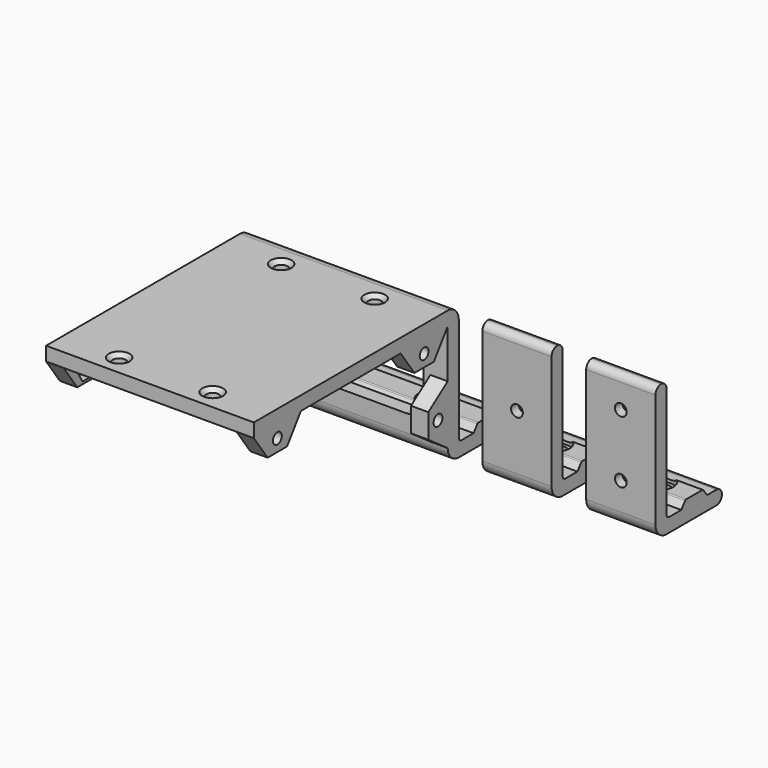
from build123d import *

# Parameters (mm, degrees)
F1_DEPTH        = 20
F2_R            = 3
F3_DEPTH        = 6
F7_D            = 3.4
F7_DEPTH        = 12
F7_CSINK_D      = 6
F7_CSINK_ANGLE  = 90
F7_TIP          = 1.0214630523
F10_DEPTH       = 20
F11_R           = 3
F12_DEPTH       = 12.5
F13_R           = 4
F14_DEPTH       = 2
F16_D           = 3.4
F16_DEPTH       = 12
F16_CSINK_D     = 6
F16_CSINK_ANGLE = 90
F16_TIP         = 1.0214630523
F19_DEPTH       = 60
F20_W           = 60
F20_H           = 70
F21_DEPTH       = 4
F22_R           = 4
F24_D           = 5.7
F25_R           = 2.85
F26_DEPTH       = 2
F28_D           = 3.7
F28_CSINK_D     = 6
F28_CSINK_ANGLE = 90
F4_R            = 4
F29_DEPTH       = 2
F31_DEPTH       = 25
F33_DEPTH       = 5
F32_R           = 1.6
F34_DEPTH       = 2.5
F40_ANGLE       = 90


with BuildPart() as f1:
    # F0 (on Right) → F1 (new body)
    with BuildSketch(Plane.YZ):
        with BuildLine():
            Line((5.35, 0), (1, 0))
            ThreePointArc((1, 0), (0.2928932188, 0.2928932188), (0, 1))
            Line((0, 1), (0, 33))
            ThreePointArc((0, 33), (-0.5857864376, 34.4142135624), (-2, 35))
            ThreePointArc((-2, 35), (-3.4142135624, 34.4142135624), (-4, 33))
            Line((-4, 33), (-4, 0))
            ThreePointArc((-4, 0), (-2.8284271247, -2.8284271247), (0, -4))
            Line((0, -4), (18, -4))
            ThreePointArc((18, -4), (19.4142135624, -3.4142135624), (20, -2))
            ThreePointArc((20, -2), (19.4142135624, -0.5857864376), (18, 0))
            Line((18, 0), (14.65, 0))
            Line((14.65, 0), (5.35, 0))
        make_face()
        with BuildLine():
            Line((6.7, 1.8), (5.35, 0))
            Line((5.35, 0), (14.65, 0))
            Line((14.65, 0), (13.3, 1.8))
            ThreePointArc((13.3, 1.8), (13.1236067977, 1.9472135955), (12.9, 2))
            Line((12.9, 2), (10, 2))
            Line((10, 2), (7.1, 2))
            ThreePointArc((7.1, 2), (6.8763932023, 1.9472135955), (6.7, 1.8))
        make_face()
    extrude(amount=F1_DEPTH)

    # F2 (on face) → F3 (cut, through all)
    with BuildSketch(Plane(origin=(0, 0, -4), x_dir=(1, 0, 0), z_dir=(0, 0, -1))):
        with Locations((10, -10)):
            Circle(F2_R)
    extrude(amount=-F3_DEPTH, mode=Mode.SUBTRACT)

    # F7
    with Locations(Plane(origin=(0, 0, 0), x_dir=(-1, 0, 0), z_dir=(0, 1, 0))):
        with Locations((-10, 26), (-10, 8)):
            CounterSinkHole(F7_D / 2, F7_CSINK_D / 2, depth=F7_DEPTH, counter_sink_angle=F7_CSINK_ANGLE)
            with Locations((0, 0, -(F7_DEPTH + F7_TIP / 2))):  # 118° drill point
                Cone(0, F7_D / 2, F7_TIP, mode=Mode.SUBTRACT)

    # F4 (on face) → F29 (cut)
    with BuildSketch(Plane.XY.offset(2)):
        with Locations((10, 10)):
            Circle(F4_R)
    extrude(amount=-F29_DEPTH, mode=Mode.SUBTRACT)


with BuildPart() as f10:
    # F9 (on offset) → F10 (new body)
    with BuildSketch(Plane.YZ.offset(-10)):
        with BuildLine():
            ThreePointArc((1, 0), (0.2928932188, 0.2928932188), (0, 1))
            Line((0, 1), (0, 33))
            ThreePointArc((0, 33), (-0.5857864376, 34.4142135624), (-2, 35))
            ThreePointArc((-2, 35), (-3.4142135624, 34.4142135624), (-4, 33))
            Line((-4, 33), (-4, 0))
            ThreePointArc((-4, 0), (-2.8284271247, -2.8284271247), (0, -4))
            Line((0, -4), (18, -4))
            ThreePointArc((18, -4), (19.4142135624, -3.4142135624), (20, -2))
            ThreePointArc((20, -2), (19.4142135624, -0.5857864376), (18, 0))
            Line((18, 0), (14.65, 0))
            Line((14.65, 0), (5.35, 0))
            Line((5.35, 0), (1, 0))
        make_face()
        with BuildLine():
            Line((6.7, 1.8), (5.35, 0))
            Line((5.35, 0), (14.65, 0))
            Line((14.65, 0), (13.3, 1.8))
            ThreePointArc((13.3, 1.8), (13.1236067977, 1.9472135955), (12.9, 2))
            Line((12.9, 2), (10, 2))
            Line((10, 2), (7.1, 2))
            ThreePointArc((7.1, 2), (6.8763932023, 1.9472135955), (6.7, 1.8))
        make_face()
    extrude(amount=-F10_DEPTH)

    # F11 (on face) → F12 (cut, symmetric)
    with BuildSketch(Plane.XY):
        with Locations((-20, 10)):
            Circle(F11_R)
    extrude(amount=F12_DEPTH, both=True, mode=Mode.SUBTRACT)

    # F13 (on face) → F14 (cut)
    with BuildSketch(Plane.XY.offset(2)):
        with Locations((-20, 10)):
            Circle(F13_R)
    extrude(amount=-F14_DEPTH, mode=Mode.SUBTRACT)

    # F16
    with Locations(Plane(origin=(0, 0, 0), x_dir=(-1, 0, 0), z_dir=(0, 1, 0))):
        with Locations((20, 16)):
            CounterSinkHole(F16_D / 2, F16_CSINK_D / 2, depth=F16_DEPTH, counter_sink_angle=F16_CSINK_ANGLE)
            with Locations((0, 0, -(F16_DEPTH + F16_TIP / 2))):  # 118° drill point
                Cone(0, F16_D / 2, F16_TIP, mode=Mode.SUBTRACT)


with BuildPart() as f19:
    # F18 (on offset) → F19 (new body)
    with BuildSketch(Plane.YZ.offset(-40)):
        with BuildLine():
            Line((0, 35.0000039041), (-4, 35.0000039041))
            Line((-4, 35.0000039041), (-4, 0))
            ThreePointArc((-4, 0), (-2.8284271247, -2.8284271247), (0, -4))
            Line((0, -4), (18, -4))
            ThreePointArc((18, -4), (19.4142135624, -3.4142135624), (20, -2))
            ThreePointArc((20, -2), (19.4142135624, -0.5857864376), (18, 0))
            Line((18, 0), (14.65, 0))
            Line((14.65, 0), (5.35, 0))
            Line((5.35, 0), (1, 0))
            ThreePointArc((1, 0), (0.2928932188, 0.2928932188), (0, 1))
            Line((0, 1), (0, 35.0000039041))
        make_face()
        with BuildLine():
            Line((6.7, 1.8), (5.35, 0))
            Line((5.35, 0), (14.65, 0))
            Line((14.65, 0), (13.3, 1.8))
            ThreePointArc((13.3, 1.8), (13.1236067977, 1.9472135955), (12.9, 2))
            Line((12.9, 2), (10, 2))
            Line((10, 2), (7.1, 2))
            ThreePointArc((7.1, 2), (6.8763932023, 1.9472135955), (6.7, 1.8))
        make_face()
    extrude(amount=-F19_DEPTH)

    # F20 (on face) → F21 (join)
    with BuildSketch(Plane.XY.offset(35.0000039041)):
        with Locations((-70, -39)):
            Rectangle(F20_W, F20_H)
    extrude(amount=-F21_DEPTH)

    # F22
    f22_edges = [f19.edges().sort_by_distance(p)[0] for p in [
        (-70, 0, 35.000004),
    ]]
    fillet(f22_edges, radius=F22_R)

    # F24 (through all)
    with Locations(Plane(origin=(0, 0, -4), x_dir=(1, 0, 0), z_dir=(0, 0, -1))):
        with Locations((-85, -10), (-55, -10)):
            Hole(F24_D / 2)

    # F25 (on face) → F26 (cut, through all)
    with BuildSketch(Plane.XY.offset(2)):
        with BuildLine():
            ThreePointArc((-81.5590698932, 7.1), (-80.7730516042, 8.4563331772), (-80.5, 10))
            ThreePointArc((-80.5, 10), (-80.7730516042, 11.5436668228), (-81.5590698932, 12.9))
            Line((-81.5590698932, 12.9), (-88.4409301068, 12.9))
            ThreePointArc((-88.4409301068, 12.9), (-89.5, 10), (-88.4409301068, 7.1))
            Line((-88.4409301068, 7.1), (-81.5590698932, 7.1))
        make_face()
        with Locations((-85, 10)):
            Circle(F25_R, mode=Mode.SUBTRACT)
        with BuildLine():
            Line((-51.5590698932, 12.9), (-58.4409301068, 12.9))
            ThreePointArc((-58.4409301068, 12.9), (-59.5, 10), (-58.4409301068, 7.1))
            Line((-58.4409301068, 7.1), (-51.5590698932, 7.1))
            ThreePointArc((-51.5590698932, 7.1), (-50.7730516042, 8.4563331772), (-50.5, 10))
            ThreePointArc((-50.5, 10), (-50.7730516042, 11.5436668228), (-51.5590698932, 12.9))
        make_face()
        with Locations((-55, 10)):
            Circle(F25_R, mode=Mode.SUBTRACT)
        with Locations((-55, 10)):
            Circle(F25_R)
        with BuildLine():
            Line((-88.4409301068, 12.9), (-81.5590698932, 12.9))
            ThreePointArc((-81.5590698932, 12.9), (-85, 14.5), (-88.4409301068, 12.9))
        make_face()
        with BuildLine():
            ThreePointArc((-88.4409301068, 7.1), (-85, 5.5), (-81.5590698932, 7.1))
            Line((-81.5590698932, 7.1), (-88.4409301068, 7.1))
        make_face()
        with BuildLine():
            ThreePointArc((-51.5590698932, 12.9), (-55, 14.5), (-58.4409301068, 12.9))
            Line((-58.4409301068, 12.9), (-51.5590698932, 12.9))
        make_face()
        with BuildLine():
            Line((-51.5590698932, 7.1), (-58.4409301068, 7.1))
            ThreePointArc((-58.4409301068, 7.1), (-55, 5.5), (-51.5590698932, 7.1))
        make_face()
    extrude(amount=-F26_DEPTH, mode=Mode.SUBTRACT)

    # F28 (through all)
    with Locations(Plane.XY.offset(35.0000039041)):
        with Locations((-83.5, -9.75), (-83.5, -68.25), (-56.5, -68.25), (-56.5, -9.75)):
            CounterSinkHole(F28_D / 2, F28_CSINK_D / 2, counter_sink_angle=F28_CSINK_ANGLE)

    # F30 (on face) → F31 (cut)
    with BuildSketch(Plane.XZ.offset(4)):
        with BuildLine():
            Line((-88, 5), (-52, 5))
            ThreePointArc((-52, 5), (-48.4644660941, 6.4644660941), (-47, 10))
            Line((-47, 10), (-47, 20.0000039041))
            ThreePointArc((-47, 20.0000039041), (-48.4644660941, 23.53553781), (-52, 25.0000039041))
            Line((-52, 25.0000039041), (-88, 25.0000039041))
            ThreePointArc((-88, 25.0000039041), (-91.5355339059, 23.53553781), (-93, 20.0000039041))
            Line((-93, 20.0000039041), (-93, 10))
            ThreePointArc((-93, 10), (-91.5355339059, 6.4644660941), (-88, 5))
        make_face()
    extrude(amount=-F31_DEPTH, mode=Mode.SUBTRACT)


with BuildPart() as f33:
    # F32 (on face) → F33 (new body)
    with BuildSketch(Plane(origin=(-100, 0, 0), x_dir=(0, -1, 0), z_dir=(-1, 0, 0))):
        Polygon((69, 24.0000039041), (74, 31.0000039041), (57, 31.0000039041), (62, 24.0000039041), align=None)
        Polygon((68.7331615075, 27.5000039041), (67.1165807537, 24.7000039041), (63.8834192463, 24.7000039041), (62.2668384925, 27.5000039041), (63.8834192463, 30.3000039041), (67.1165807537, 30.3000039041), align=None, mode=Mode.SUBTRACT)
    extrude(amount=-F33_DEPTH)

    # F32 (on face) → F34 (join)
    with BuildSketch(Plane(origin=(-100, 0, 0), x_dir=(0, -1, 0), z_dir=(-1, 0, 0))):
        Polygon((63.8834192463, 24.7000039041), (67.1165807537, 24.7000039041), (68.7331615075, 27.5000039041), (67.1165807537, 30.3000039041), (63.8834192463, 30.3000039041), (62.2668384925, 27.5000039041), align=None)
        with Locations((65.5, 27.5000039041)):
            Circle(F32_R, mode=Mode.SUBTRACT)
    extrude(amount=-F34_DEPTH)


with BuildPart() as f36_1:
    # F36: instance of F33
    add(f33.part.mirror(Plane(origin=(-70, -19.678374032, 21.8068336771), x_dir=(0, -1, 0), z_dir=(-1, 0, 0))))


with BuildPart() as f38_1:
    # F38: instance of F36_1
    add(f36_1.part.mirror(Plane(origin=(-70, -39, 24.4836423341), x_dir=(1, 0, 0), z_dir=(0, -1, 0))))


with BuildPart() as f38_2:
    # F38: instance of F33
    add(f33.part.mirror(Plane(origin=(-70, -39, 24.4836423341), x_dir=(1, 0, 0), z_dir=(0, -1, 0))))


with BuildPart() as f39_1:
    # F39: copy of F38_2
    add(f38_2.part.moved(Location((0, 0, -31.0000039041))))


with BuildPart() as f39_2:
    # F39: copy of F38_1
    add(f38_1.part.moved(Location((0, 0, -31.0000039041))))


with BuildPart() as f39_2_1:
    # F40: moved
    add(f39_2.part.rotate(Axis((-97.5, -4, 0), (-1, 0, 0)), F40_ANGLE))


with BuildPart() as f39_1_1:
    # F40: moved
    add(f39_1.part.rotate(Axis((-97.5, -4, 0), (-1, 0, 0)), F40_ANGLE))


with BuildPart() as f19_1:
    add(f19.part)

    # F41: union F39_2, F39_1, F38_2, F38_1, F36_1, F33
    add(f39_2_1.part)
    add(f39_1_1.part)
    add(f38_2.part)
    add(f38_1.part)
    add(f36_1.part)
    add(f33.part)


solid = Compound([f1.part, f10.part, f19_1.part])
